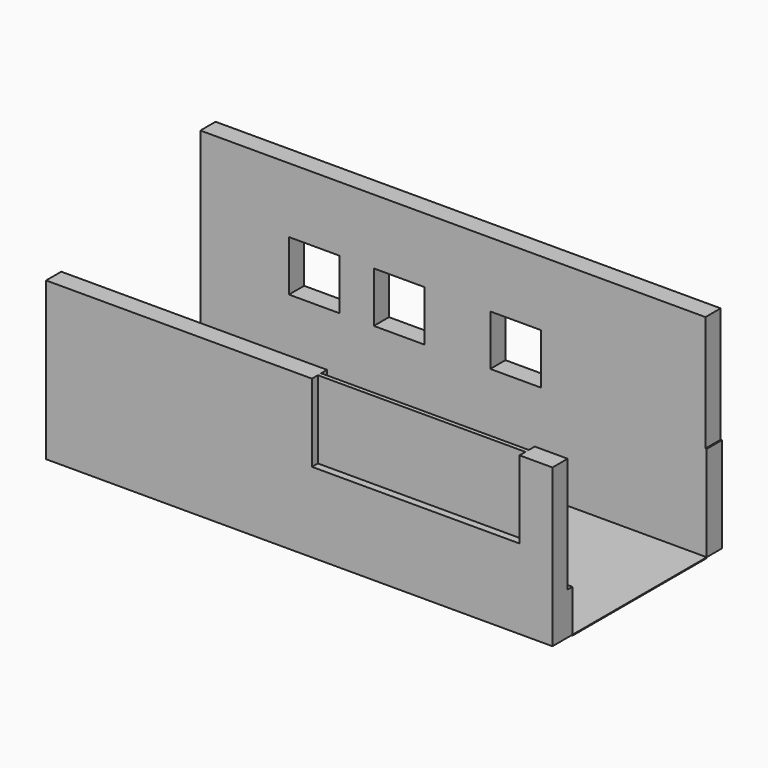
from build123d import *

# Parameters (mm, degrees)
F1_W      = 600
F1_H      = 22.5
F2_DEPTH  = 113
F3_W      = 105
F3_H      = 22.5
F4_DEPTH  = 137
F5_W      = 22.5
F5_H      = 77
F6_DEPTH  = 100.5
F7_W      = 40.5
F7_H      = 22.5
F8_DEPTH  = 61
F9_W      = 22.5
F9_H      = 77
F10_DEPTH = 138
F11_W     = 78
F11_H     = 22.5
F12_DEPTH = 61
F13_W     = 22.5
F13_H     = 77
F14_DEPTH = 60
F15_W     = 195
F15_H     = 22.5
F16_DEPTH = 140
F0_W      = 600
F0_H      = 199
F17_DEPTH = 1
F18_W     = 600
F18_H     = 29.5
F19_DEPTH = 50
F20_W     = 600
F20_H     = 22.5
F21_DEPTH = 136.5
F23_START = -315
F22_W     = 22.5
F22_H     = 92
F23_DEPTH = 246
F24_W     = 246
F24_H     = 5
F25_DEPTH = 92
F26_DEPTH = 8.75
F27_DEPTH = 8.75


with BuildPart() as f2:
    # F1 (on face) → F2 (new body)
    with BuildSketch(Plane.XY):
        with Locations((300, 11.25)):
            Rectangle(F1_W, F1_H)
    extrude(amount=F2_DEPTH)

    # F3 (on face) → F4 (join)
    with BuildSketch(Plane.XY.offset(113)):
        with Locations((52.5, 11.25)):
            Rectangle(F3_W, F3_H)
    extrude(amount=F4_DEPTH)

    # F5 (on face) → F6 (join)
    with BuildSketch(Plane.YZ.offset(105)):
        with Locations((11.25, 211.5)):
            Rectangle(F5_W, F5_H)
    extrude(amount=F6_DEPTH)

    # F7 (on face) → F8 (join)
    with BuildSketch(Plane(origin=(0, 0, 173), x_dir=(1, 0, 0), z_dir=(0, 0, -1))):
        with Locations((185.25, -11.25)):
            Rectangle(F7_W, F7_H)
    extrude(amount=F8_DEPTH)

    # F9 (on face) → F10 (join)
    with BuildSketch(Plane.YZ.offset(205.5)):
        with Locations((11.25, 211.5)):
            Rectangle(F9_W, F9_H)
    extrude(amount=F10_DEPTH)

    # F11 (on face) → F12 (join)
    with BuildSketch(Plane(origin=(0, 0, 173), x_dir=(1, 0, 0), z_dir=(0, 0, -1))):
        with Locations((304.5, -11.25)):
            Rectangle(F11_W, F11_H)
    extrude(amount=F12_DEPTH)

    # F13 (on face) → F14 (join)
    with BuildSketch(Plane.YZ.offset(343.5)):
        with Locations((11.25, 211.5)):
            Rectangle(F13_W, F13_H)
    extrude(amount=F14_DEPTH)

    # F15 (on face) → F16 (join)
    with BuildSketch(Plane.XY.offset(250)):
        with Locations((501, 11.25)):
            Rectangle(F15_W, F15_H)
    extrude(amount=-F16_DEPTH)


with BuildPart() as f17:
    # F0 (on Top) → F17 (new body)
    with BuildSketch(Plane.XY):
        with Locations((300, -99.5)):
            Rectangle(F0_W, F0_H)
    extrude(amount=-F17_DEPTH)


with BuildPart() as f19:
    # F18 (on face) → F19 (new body)
    with BuildSketch(Plane.XY):
        with Locations((300, -213.75)):
            Rectangle(F18_W, F18_H)
    extrude(amount=F19_DEPTH)

    # F20 (on face) → F21 (join)
    with BuildSketch(Plane.XY.offset(50)):
        with Locations((300, -217.25)):
            Rectangle(F20_W, F20_H)
    extrude(amount=F21_DEPTH)

    # F22 (on face) → F23 (cut)
    with BuildSketch(Plane(origin=(0, 0, 0), x_dir=(0, -1, 0), z_dir=(-1, 0, 0)).offset(F23_START)):
        with Locations((217.25, 140.5)):
            Rectangle(F22_W, F22_H)
    extrude(amount=-F23_DEPTH, mode=Mode.SUBTRACT)


with BuildPart() as f25:
    # F24 (on face) → F25 (new body)
    with BuildSketch(Plane.XY.offset(94.5)):
        with Locations((438, -226)):
            Rectangle(F24_W, F24_H)
    extrude(amount=F25_DEPTH)

    # F26 (add): a face of the model
    f26_faces = [f25.faces().sort_by_distance(p)[0] for p in [
        (438, -223.5, 140.5),
    ]]
    extrude(f26_faces, amount=F26_DEPTH)

    # F27 (cut): a face of the model
    f27_faces = [f25.faces().sort_by_distance(p)[0] for p in [
        (438, -228.5, 140.5),
    ]]
    extrude(f27_faces, amount=-F27_DEPTH, mode=Mode.SUBTRACT)


solid = Compound([f2.part, f17.part, f19.part, f25.part])
